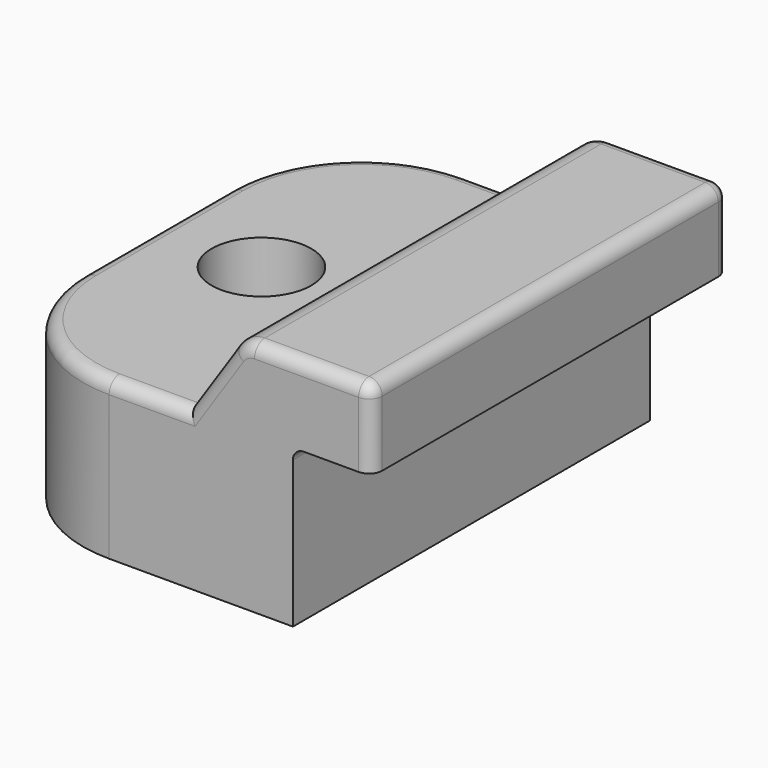
from build123d import *

# Parameters (mm, degrees)
F1_DEPTH = 17
F2_R     = 0.5
F3_R     = 1.9
F4_DEPTH = 25
F5_R     = 5
F6_R     = 0.5
F7_R     = 1
F8_R     = 0.49999


# Not quite as in the source:
# - a fillet or chamfer is up to 0.001 mm smaller than in the source, because OpenCascade refuses the exact size


with BuildPart() as f1:
    # F0 (on Front) → F1 (new body)
    with BuildSketch(Plane.XZ):
        with BuildLine():
            Line((-12, 0), (0, 0))
            Line((0, 0), (0, 5.58898558))
            ThreePointArc((0, 5.58898558), (0.1203833365, 5.8796166635), (0.41101442, 6))
            Line((0.41101442, 6), (3, 6))
            Line((3, 6), (3, 9))
            Line((3, 9), (-2, 9))
            Line((-2, 9), (-4, 6))
            Line((-4, 6), (-12, 6))
            Line((-12, 6), (-12, 0))
        make_face()
    extrude(amount=F1_DEPTH)

    # F2
    f2_edges = [f1.edges().sort_by_distance(p)[0] for p in [
        (3, -8.5, 9),
    ]]
    fillet(f2_edges, radius=F2_R)

    # F3 (on face) → F4 (cut)
    with BuildSketch(Plane.XY.offset(6)):
        with Locations((-8, -8.5)):
            Circle(F3_R)
    extrude(amount=-F4_DEPTH, mode=Mode.SUBTRACT)

    # F5
    f5_edges = [f1.edges().sort_by_distance(p)[0] for p in [
        (-12, -17, 3),
        (-12, 0, 3),
    ]]
    fillet(f5_edges, radius=F5_R)

    # F6
    f6_edges = [f1.edges().sort_by_distance(p)[0] for p in [
        (-10.535534, -15.535534, 6),
    ]]
    fillet(f6_edges, radius=F6_R)

    # F7
    f7_edges = [f1.edges().sort_by_distance(p)[0] for p in [
        (-2, -8.5, 9),
    ]]
    fillet(f7_edges, radius=F7_R)

    # F8 (radius 0.5 in the source; OpenCascade refuses exactly that, so slightly less here)
    f8_edges = [f1.edges().sort_by_distance(p)[0] for p in [
        (-3.148433, -17, 7.27735),
        (-3.148433, 0, 7.27735),
    ]]
    fillet(f8_edges, radius=F8_R)


solid = f1.part
